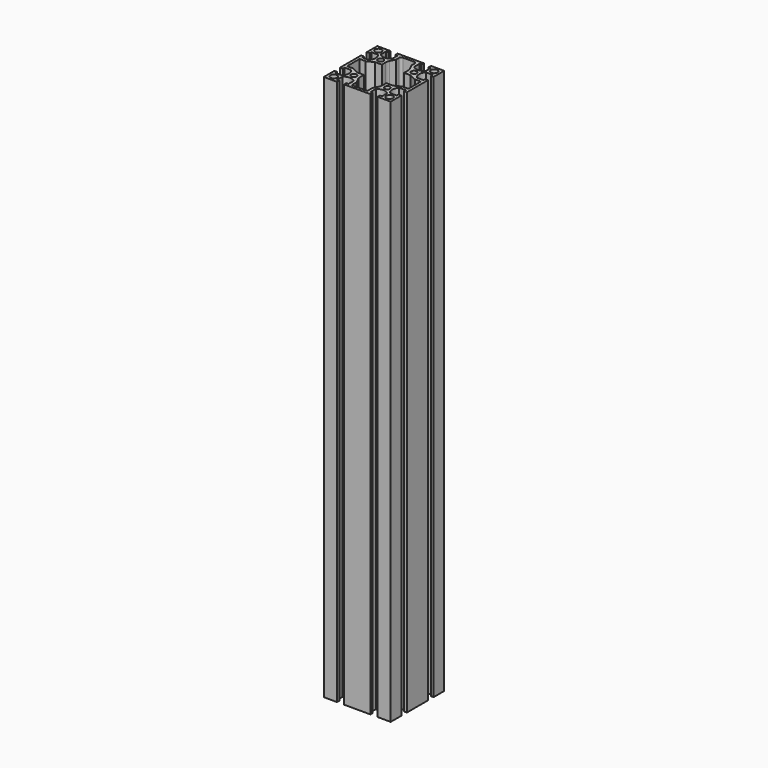
from build123d import *

# Parameters (mm, degrees)
F0_R     = 3
F0_R_2   = 2.5
F1_DEPTH = 490
F2_R     = 2
F3_R     = 7


# Not quite as in the source:
# - a feature names something its author has since deleted; it is built from what else it names


with BuildPart() as f1:
    # F0 (on Top) → F1 (new body)
    with BuildSketch(Plane.XY):
        with BuildLine():
            Line((18.15, -30), (30, -30))
            Line((30, -30), (30, -18.15))
            Line((30, -18.15), (27.5, -18.15))
            Line((27.5, -18.15), (27.5, -20.15))
            Line((27.5, -20.15), (21.5477069044, -20.15))
            ThreePointArc((21.5477069044, -20.15), (19.5, -15), (21.5477069044, -9.85))
            Line((21.5477069044, -9.85), (27.5, -9.85))
            Line((27.5, -9.85), (27.5, -11.85))
            Line((27.5, -11.85), (30, -11.85))
            Line((30, -11.85), (30, 11.85))
            Line((30, 11.85), (27.5, 11.85))
            Line((27.5, 11.85), (27.5, 9.85))
            Line((27.5, 9.85), (21.5477069044, 9.85))
            ThreePointArc((21.5477069044, 9.85), (19.5, 15), (21.5477069044, 20.15))
            Line((21.5477069044, 20.15), (27.5, 20.15))
            Line((27.5, 20.15), (27.5, 18.15))
            Line((27.5, 18.15), (30, 18.15))
            Line((30, 18.15), (30, 30))
            Line((30, 30), (18.15, 30))
            Line((18.15, 30), (18.15, 27.5))
            Line((18.15, 27.5), (20.15, 27.5))
            Line((20.15, 27.5), (20.15, 21.5477069044))
            ThreePointArc((20.15, 21.5477069044), (15, 19.5), (9.85, 21.5477069044))
            Line((9.85, 21.5477069044), (9.85, 27.5))
            Line((9.85, 27.5), (11.85, 27.5))
            Line((11.85, 27.5), (11.85, 30))
            Line((11.85, 30), (-11.85, 30))
            Line((-11.85, 30), (-11.85, 27.5))
            Line((-11.85, 27.5), (-9.85, 27.5))
            Line((-9.85, 27.5), (-9.85, 21.5477069044))
            ThreePointArc((-9.85, 21.5477069044), (-15, 19.5), (-20.15, 21.5477069044))
            Line((-20.15, 21.5477069044), (-20.15, 27.5))
            Line((-20.15, 27.5), (-18.15, 27.5))
            Line((-18.15, 27.5), (-18.15, 30))
            Line((-18.15, 30), (-30, 30))
            Line((-30, 30), (-30, 18.15))
            Line((-30, 18.15), (-27.5, 18.15))
            Line((-27.5, 18.15), (-27.5, 20.15))
            Line((-27.5, 20.15), (-21.5477069044, 20.15))
            ThreePointArc((-21.5477069044, 20.15), (-19.5, 15), (-21.5477069044, 9.85))
            Line((-21.5477069044, 9.85), (-27.5, 9.85))
            Line((-27.5, 9.85), (-27.5, 11.85))
            Line((-27.5, 11.85), (-30, 11.85))
            Line((-30, 11.85), (-30, -11.85))
            Line((-30, -11.85), (-27.5, -11.85))
            Line((-27.5, -11.85), (-27.5, -9.85))
            Line((-27.5, -9.85), (-21.5477069044, -9.85))
            ThreePointArc((-21.5477069044, -9.85), (-19.5, -15), (-21.5477069044, -20.15))
            Line((-21.5477069044, -20.15), (-27.5, -20.15))
            Line((-27.5, -20.15), (-27.5, -18.15))
            Line((-27.5, -18.15), (-30, -18.15))
            Line((-30, -18.15), (-30, -30))
            Line((-30, -30), (-18.15, -30))
            Line((-18.15, -30), (-18.15, -27.5))
            Line((-18.15, -27.5), (-20.15, -27.5))
            Line((-20.15, -27.5), (-20.15, -21.5477069044))
            ThreePointArc((-20.15, -21.5477069044), (-15, -19.5), (-9.85, -21.5477069044))
            Line((-9.85, -21.5477069044), (-9.85, -27.5))
            Line((-9.85, -27.5), (-11.85, -27.5))
            Line((-11.85, -27.5), (-11.85, -30))
            Line((-11.85, -30), (11.85, -30))
            Line((11.85, -30), (11.85, -27.5))
            Line((11.85, -27.5), (9.85, -27.5))
            Line((9.85, -27.5), (9.85, -21.5477069044))
            ThreePointArc((9.85, -21.5477069044), (15, -19.5), (20.15, -21.5477069044))
            Line((20.15, -21.5477069044), (20.15, -27.5))
            Line((20.15, -27.5), (18.15, -27.5))
            Line((18.15, -27.5), (18.15, -30))
        make_face()
        with Locations((-25, -25)):
            Circle(F0_R, mode=Mode.SUBTRACT)
        with Locations((-15, -15)):
            Circle(F0_R_2, mode=Mode.SUBTRACT)
        with Locations((25, -25)):
            Circle(F0_R, mode=Mode.SUBTRACT)
        with Locations((15, -15)):
            Circle(F0_R_2, mode=Mode.SUBTRACT)
        with Locations((-25, 25)):
            Circle(F0_R, mode=Mode.SUBTRACT)
        with Locations((-15, 15)):
            Circle(F0_R_2, mode=Mode.SUBTRACT)
        Polygon((-7, 22), (-7, 27.5), (0, 27.5), (7, 27.5), (7, 22), (10, 16), (10, 10), (16, 10), (22, 7), (27.5, 7), (27.5, 0), (27.5, -7), (22, -7), (16, -10), (10, -10), (10, -16), (7, -22), (7, -27.5), (0, -27.5), (-7, -27.5), (-7, -22), (-10, -16), (-10, -10), (-16, -10), (-22, -7), (-27.5, -7), (-27.5, 0), (-27.5, 7), (-22, 7), (-16, 10), (-10, 10), (-10, 16), align=None, mode=Mode.SUBTRACT)
        with Locations((15, 15)):
            Circle(F0_R_2, mode=Mode.SUBTRACT)
        with Locations((25, 25)):
            Circle(F0_R, mode=Mode.SUBTRACT)
    extrude(amount=F1_DEPTH)

    # F2
    f2_edges = [f1.edges().sort_by_distance(p)[0] for p in [
        (-7, 27.5, 245),
        (7, 27.5, 245),
    ]]
    fillet(f2_edges, radius=F2_R)

    # F3
    f3_edges = [f1.edges().sort_by_distance(p)[0] for p in [
        (-10, 16, 245),
        (10, 16, 245),
    ]]
    fillet(f3_edges, radius=F3_R)


solid = f1.part
